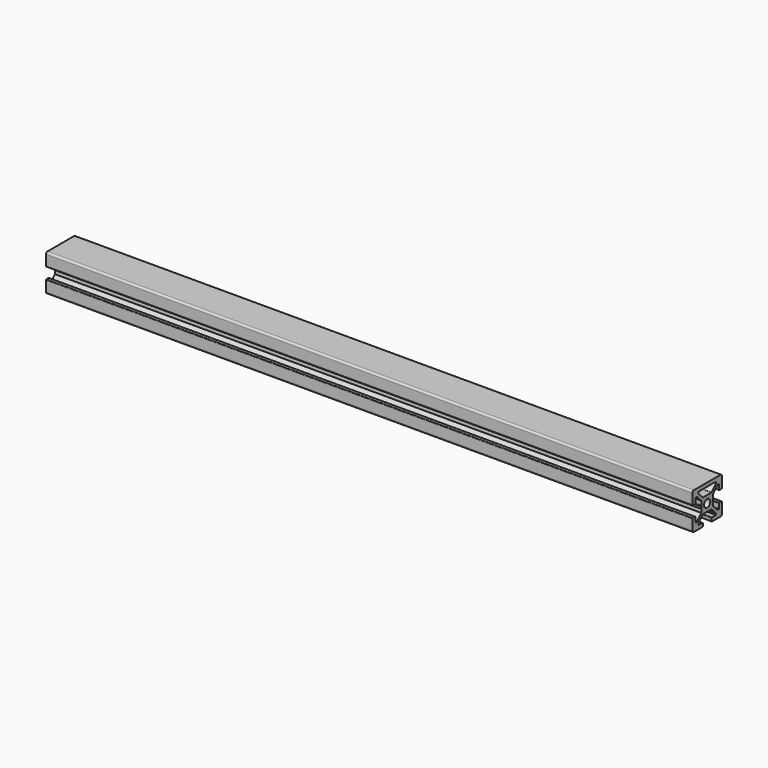
from build123d import *

# Parameters (mm, degrees)
F1_DEPTH = 175.5


# Not quite as in the source:
# - ends of sketch curves that miss each other by under 0.0002 mm in the source are joined


with BuildPart() as f1:
    # F0 (on Right) → F1 (new body, symmetric)
    with BuildSketch(Plane.YZ):
        with BuildLine():
            Line((9.043565, 10.073321), (0.043565, 10.073321))
            Line((0.043565, 10.073321), (-8.956435, 10.073321))
            ThreePointArc((-8.956435, 10.073321), (-9.6635417812, 9.7804277812), (-9.956435, 9.073321))
            Line((-9.956435, 9.073321), (-9.956435, 3.373321))
            ThreePointArc((-9.956435, 3.373321), (-9.8685670344, 3.1611889656), (-9.656435, 3.073321))
            Line((-9.656435, 3.073321), (-8.256435, 3.073321))
            ThreePointArc((-8.256435, 3.073321), (-8.0443029656, 3.1611889656), (-7.956435, 3.373321))
            Line((-7.956435, 3.373321), (-7.956435, 6.073321))
            Line((-7.956435, 6.073321), (-7.017095, 6.073321))
            Line((-7.017095, 6.073321), (-3.956435, 3.012661))
            Line((-3.956435, 3.012661), (-3.956435, 0.726911))
            ThreePointArc((-3.956435, 0.726911), (-3.9393979324, 0.5975015494), (-3.8894477764, 0.4769111291))
            Line((-3.8894477764, 0.4769111291), (-3.656435, 0.073321))
            Line((-3.656435, 0.073321), (-3.889448, -0.330269))
            ThreePointArc((-3.889448, -0.330269), (-3.956435, -0.580269), (-3.8894477764, -0.8302688709))
            Line((-3.8894477764, -0.8302688709), (-3.707412, -1.145565))
            Line((-3.707412, -1.145565), (-3.956435, -2.426679))
            Line((-3.956435, -2.426679), (-3.956435, -2.866019))
            Line((-3.956435, -2.866019), (-7.017095, -5.926679))
            Line((-7.017095, -5.926679), (-7.956435, -5.926679))
            Line((-7.956435, -5.926679), (-7.956435, -3.226679))
            ThreePointArc((-7.956435, -3.226679), (-8.0443029656, -3.0145469656), (-8.256435, -2.926679))
            Line((-8.256435, -2.926679), (-9.656435, -2.926679))
            ThreePointArc((-9.656435, -2.926679), (-9.8685670344, -3.0145469656), (-9.956435, -3.226679))
            Line((-9.956435, -3.226679), (-9.956435, -8.926679))
            ThreePointArc((-9.956435, -8.926679), (-9.6635417812, -9.6337857812), (-8.956435, -9.926679))
            Line((-8.956435, -9.926679), (-3.256435, -9.926679))
            ThreePointArc((-3.256435, -9.926679), (-3.0443029656, -9.8388110344), (-2.956435, -9.626679))
            Line((-2.956435, -9.626679), (-2.956435, -8.226679))
            ThreePointArc((-2.956435, -8.226679), (-3.0443029656, -8.0145469656), (-3.256435, -7.926679))
            Line((-3.256435, -7.926679), (-5.956435, -7.926679))
            Line((-5.956435, -7.926679), (-5.956435, -6.987339))
            Line((-5.956435, -6.987339), (-2.895775, -3.926679))
            Line((-2.895775, -3.926679), (-0.610025, -3.926679))
            ThreePointArc((-0.610025, -3.926679), (-0.4806155494, -3.9096419324), (-0.3600251291, -3.8596917764))
            Line((-0.3600251291, -3.8596917764), (-0.0645959325, -3.6891257984))
            Line((-0.0645959325, -3.6891257984), (0.2217128734, -3.8544264098))
            ThreePointArc((0.2217128734, -3.8544264098), (0.3921793907, -3.9150473077), (0.5730594828, -3.9110345539))
            ThreePointArc((0.5730594828, -3.9110345539), (0.6346161199, -3.9227524708), (0.697155, -3.926679))
            Line((0.697155, -3.926679), (2.982905, -3.926679))
            Line((2.982905, -3.926679), (6.043565, -6.987339))
            Line((6.043565, -6.987339), (6.043565, -7.926679))
            Line((6.043565, -7.926679), (3.343565, -7.926679))
            ThreePointArc((3.343565, -7.926679), (3.1314329656, -8.0145469656), (3.043565, -8.226679))
            Line((3.043565, -8.226679), (3.043565, -9.626679))
            ThreePointArc((3.043565, -9.626679), (3.1314329656, -9.8388110344), (3.343565, -9.926679))
            Line((3.343565, -9.926679), (9.043565, -9.926679))
            ThreePointArc((9.043565, -9.926679), (9.7506717812, -9.6337857812), (10.043565, -8.926679))
            Line((10.043565, -8.926679), (10.043565, -3.226679))
            ThreePointArc((10.043565, -3.226679), (9.9556970344, -3.0145469656), (9.743565, -2.926679))
            Line((9.743565, -2.926679), (8.343565, -2.926679))
            ThreePointArc((8.343565, -2.926679), (8.1314329656, -3.0145469656), (8.043565, -3.226679))
            Line((8.043565, -3.226679), (8.043565, -5.926679))
            Line((8.043565, -5.926679), (7.104225, -5.926679))
            Line((7.104225, -5.926679), (4.043565, -2.866019))
            Line((4.043565, -2.866019), (4.043565, -2.426679))
            Line((4.043565, -2.426679), (3.794542, -1.145565))
            Line((3.794542, -1.145565), (3.976578, -0.830269))
            ThreePointArc((3.976578, -0.830269), (4.043565, -0.580269), (3.9765777764, -0.3302691291))
            Line((3.9765777764, -0.3302691291), (3.743565, 0.073321))
            Line((3.743565, 0.073321), (3.976578, 0.476911))
            ThreePointArc((3.976578, 0.476911), (4.0265279324, 0.5975015494), (4.043565, 0.726911))
            Line((4.043565, 0.726911), (4.043565, 3.012661))
            Line((4.043565, 3.012661), (7.104225, 6.073321))
            Line((7.104225, 6.073321), (8.043565, 6.073321))
            Line((8.043565, 6.073321), (8.043565, 3.373321))
            ThreePointArc((8.043565, 3.373321), (8.1314329656, 3.1611889656), (8.343565, 3.073321))
            Line((8.343565, 3.073321), (9.743565, 3.073321))
            ThreePointArc((9.743565, 3.073321), (9.9556970344, 3.1611889656), (10.043565, 3.373321))
            Line((10.043565, 3.373321), (10.043565, 9.073321))
            ThreePointArc((10.043565, 9.073321), (9.7506717812, 9.7804277812), (9.043565, 10.073321))
        make_face()
        with BuildLine():
            ThreePointArc((0.043565, 2.173321), (2.143565, 0.073321), (0.043565, -2.026679))
            ThreePointArc((0.043565, -2.026679), (-2.056435, 0.073321), (0.043565, 2.173321))
        make_face(mode=Mode.SUBTRACT)
        with BuildLine():
            Line((2.775798, 4.073321), (0.043565, 4.073321))
            Line((0.043565, 4.073321), (-2.688668, 4.073321))
            ThreePointArc((-2.688668, 4.073321), (-2.8800097162, 4.1113812337), (-3.0422213906, 4.2197676094))
            Line((-3.0422213906, 4.2197676094), (-5.809988, 6.987535))
            ThreePointArc((-5.809988, 6.987535), (-5.9183747663, 7.1497462838), (-5.956435, 7.341088))
            Line((-5.956435, 7.341088), (-5.956435, 7.573321))
            ThreePointArc((-5.956435, 7.573321), (-5.8099883906, 7.9268743906), (-5.456435, 8.073321))
            Line((-5.456435, 8.073321), (0.043565, 8.073321))
            Line((0.043565, 8.073321), (5.543565, 8.073321))
            ThreePointArc((5.543565, 8.073321), (5.8971183906, 7.9268743906), (6.043565, 7.573321))
            Line((6.043565, 7.573321), (6.043565, 7.341088))
            ThreePointArc((6.043565, 7.341088), (6.0055047663, 7.1497462838), (5.8971183906, 6.9875346094))
            Line((5.8971183906, 6.9875346094), (3.129351, 4.219768))
            ThreePointArc((3.129351, 4.219768), (2.9671397162, 4.1113812337), (2.775798, 4.073321))
        make_face(mode=Mode.SUBTRACT)
    extrude(amount=F1_DEPTH, both=True)


solid = f1.part
